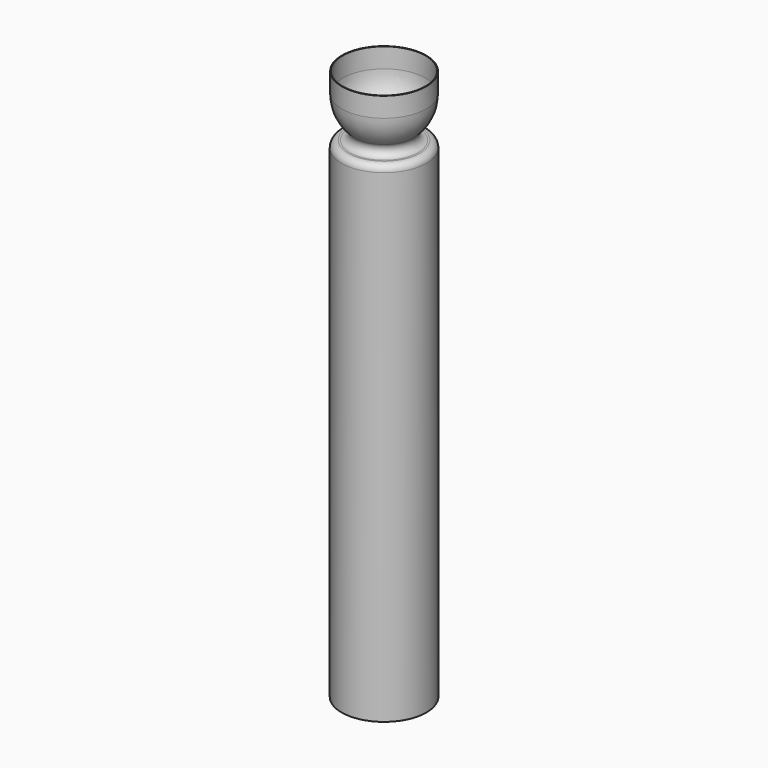
from build123d import *

# Parameters (mm, degrees)
F0_R     = 192.6943149474
F1_DEPTH = 278.8188457489
F2_R     = 188.1925897504
F3_R     = 194.2459802586
F4_DEPTH = 270.4450786114
F6_T     = -2.54
F7_DEPTH = 843.5312509537
F8_DEPTH = 1129.975438118


# Not quite as in the source:
# - a fillet or chamfer that OpenCascade refuses, or shapes differently, is made with other operations: its cross-section is extruded or revolved along the edge and cut away or added


with BuildPart() as f1:
    # F0 (on Top) → F1 (new body)
    with BuildSketch(Plane.XY):
        Circle(F0_R)
    extrude(amount=F1_DEPTH)

    # F2
    f2_edges = [f1.edges().sort_by_distance(p)[0] for p in [
        (-192.694315, 0, 0),
    ]]
    fillet(f2_edges, radius=F2_R)

    # F3 (on Top) → F4 (join)
    with BuildSketch(Plane.XY):
        Circle(F3_R)
    extrude(amount=-F4_DEPTH)

    # F5: fillet of radius 30.48 on 2 edges, made by hand

    # F5_s1 → F5_t2 (revolve)
    with BuildSketch(Plane.XZ):
        with BuildLine():
            ThreePointArc((155.9763121834, -0.0004), (127.6997450573, 19.1003639784), (134.862440304, 52.4635057638))
            Line((134.862440304, 52.4635057638), (132.7510531161, 54.6618417328))
            ThreePointArc((132.7510531161, 54.6618417328), (75.136788898, 14.3228364086), (4.501725197, 3.0480546074))
            Line((4.501725197, 3.0480546074), (4.501725197, -3.0480546074))
            ThreePointArc((4.501725197, -3.0480546074), (80.2390186902, -3.0480546074), (155.9763121834, -3.0484546074))
            Line((155.9763121834, -3.0484546074), (155.9763121834, -0.0004))
        make_face()
    revolve(axis=Axis((0, 0, 0), (0, 0, 1)))

    # F5_s3 → F5_t4 (revolve, cut)
    with BuildSketch(Plane.XZ):
        with BuildLine():
            ThreePointArc((194.2463802586, -30.4809656854), (185.3185949492, -8.9273853094), (163.7650145732, 0.0004))
            Line((163.7650145732, 0.0004), (163.7650145732, 3.0485365685))
            ThreePointArc((163.7650145732, 3.0485365685), (179.0054974159, 3.0481365685), (194.2459802586, 3.0481365685))
            Line((194.2459802586, 3.0481365685), (197.2941168272, 0))
            ThreePointArc((197.2941168272, 0), (197.2941168272, -15.2404828427), (197.2945168272, -30.4809656854))
            Line((197.2945168272, -30.4809656854), (194.2463802586, -30.4809656854))
        make_face()
    revolve(axis=Axis((0, 0, 0), (0, 0, 1)), mode=Mode.SUBTRACT)

    # F6
    f6_openings = [f1.faces().sort_by_distance(p)[0] for p in [
        (0, 0, 278.818846),
    ]]
    offset(amount=F6_T, openings=f6_openings)

    # F7 (add): a face of the model
    f7_faces = [f1.faces().sort_by_distance(p)[0] for p in [
        (0, 0, -270.4450786114),
    ]]
    extrude(f7_faces, amount=F7_DEPTH)

    # F8 (add): a face of the model
    f8_faces = [f1.faces().sort_by_distance(p)[0] for p in [
        (0, 0, -1113.976329565),
    ]]
    extrude(f8_faces, amount=F8_DEPTH)


solid = f1.part
